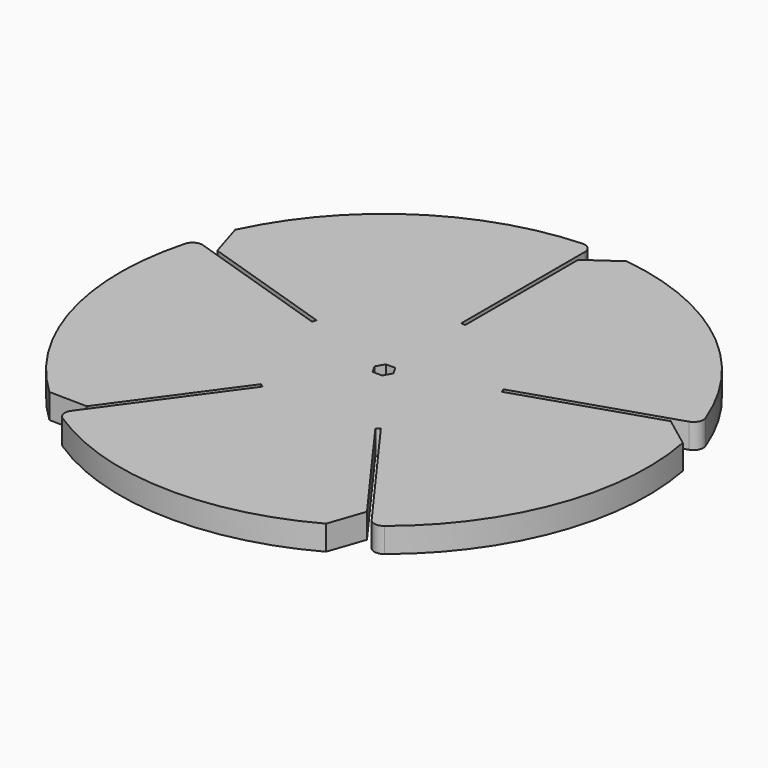
from build123d import *

# Parameters (mm, degrees)
F1_DEPTH = 19.05
F3_DEPTH = 19.05
F4_R     = 7.62


# Not quite as in the source:
# - a length typed as a fraction of an inch, garbled in the dataset ("3 / 203.2 mm" for 3/8 in), is restored


with BuildPart() as f1:
    # F0 (on Top) → F1 (new body)
    with BuildSketch(Plane.XY):
        with BuildLine():
            Line((-72.9806935994, 21.976900663), (-193.7584921492, 61.2199862795))
            ThreePointArc((-193.7584921492, 61.2199862795), (-196.6172683272, -51.3019472882), (-139.1466642939, -148.0825641859))
            Line((-139.1466642939, -148.0825641859), (-109.9986790571, -148.5913441608))
            Line((-109.9986790571, -148.5913441608), (-46.1249232824, -60.6766615198))
            Line((-46.1249232824, -60.6766615198), (-43.453549167, -62.6175284229))
            Line((-43.453549167, -62.6175284229), (-118.0983337572, -165.3572603903))
            ThreePointArc((-118.0983337572, -165.3572603903), (-11.9670260336, -202.8473078153), (97.8362036413, -178.0963707015))
            Line((97.8362036413, -178.0963707015), (107.3273049417, -150.5322110638))
            Line((107.3273049417, -150.5322110638), (43.453549167, -62.6175284229))
            Line((43.453549167, -62.6175284229), (46.1249232824, -60.6766615198))
            Line((46.1249232824, -60.6766615198), (120.7697078726, -163.4163934872))
            ThreePointArc((120.7697078726, -163.4163934872), (189.2212394942, -74.064583468), (199.6127634745, 38.0129538194))
            Line((199.6127634745, 38.0129538194), (176.330601432, 55.5573213216))
            Line((176.330601432, 55.5573213216), (72.9806935994, 21.976900663))
            Line((72.9806935994, 21.976900663), (71.960319484, 25.1172892798))
            Line((71.960319484, 25.1172892798), (192.7381180338, 64.3603748963))
            ThreePointArc((192.7381180338, 64.3603748963), (128.9121834343, 157.0728778695), (25.5312687742, 201.5896681747))
            Line((25.5312687742, 201.5896681747), (1.651, 184.8685239645))
            Line((1.651, 184.8685239645), (1.651, 76.2))
            Line((1.651, 76.2), (-1.651, 76.2))
            Line((-1.651, 76.2), (-1.651, 203.1932927018))
            ThreePointArc((-1.651, 203.1932927018), (-109.5491285678, 171.1409607021), (-183.8335715961, 86.5763128934))
            Line((-183.8335715961, 86.5763128934), (-175.3102273166, 58.6977099385))
            Line((-175.3102273166, 58.6977099385), (-71.960319484, 25.1172892798))
            Line((-71.960319484, 25.1172892798), (-72.9806935994, 21.976900663))
        make_face()
    extrude(amount=F1_DEPTH)

    # F2 (on face) → F3 (cut, through all)
    with BuildSketch(Plane.XY.offset(19.05)):
        Polygon((3.6661742094, 6.35), (-3.6661742094, 6.35), (-7.3323484187, 0), (-3.6661742094, -6.35), (3.6661742094, -6.35), (7.3323484187, 0), align=None)
    extrude(amount=-F3_DEPTH, mode=Mode.SUBTRACT)

    # F4
    f4_edges = [f1.edges().sort_by_distance(p)[0] for p in [
        (-193.758492, 61.219986, 9.525),
        (-1.651, 203.193293, 9.525),
        (192.738118, 64.360375, 9.525),
        (120.769708, -163.416393, 9.525),
        (-118.098334, -165.35726, 9.525),
    ]]
    fillet(f4_edges, radius=F4_R)


solid = f1.part
